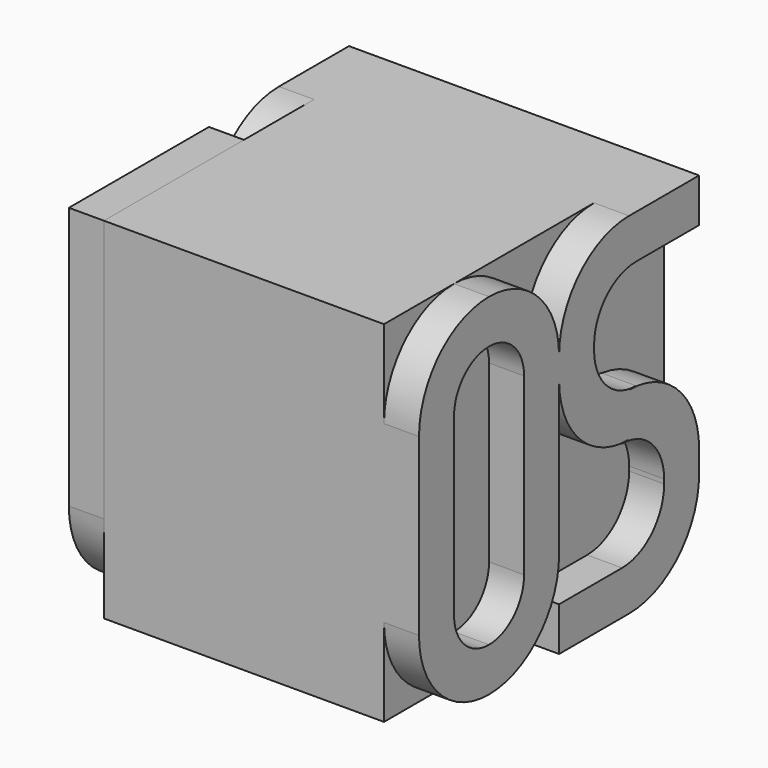
from build123d import *

# Parameters (mm, degrees)
F3_DEPTH = 2.54
F4_DEPTH = 2.54
F5_W     = 25.4
F5_H     = 25.4
F6_DEPTH = 20.32


with BuildPart() as f3:
    # F0 (on Right) → F3 (new body)
    with BuildSketch(Plane.YZ):
        with BuildLine():
            Line((0, 4.7625), (0, 6.35))
            ThreePointArc((0, 6.35), (-1.8598719395, 10.8401280605), (-6.35, 12.7))
            ThreePointArc((-6.35, 12.7), (-10.8401280605, 10.8401280605), (-12.7, 6.35))
            Line((-12.7, 6.35), (-12.7, -6.35))
            ThreePointArc((-12.7, -6.35), (-10.8401280605, -10.8401280605), (-6.35, -12.7))
            ThreePointArc((-6.35, -12.7), (-1.8598719395, -10.8401280605), (0, -6.35))
            Line((0, -6.35), (0, -3.81))
            Line((0, -3.81), (0, 4.7625))
        make_face()
        with BuildLine():
            ThreePointArc((-6.35, 9.525), (-4.1049359697, 8.5950640303), (-3.175, 6.35))
            Line((-3.175, 6.35), (-3.175, -6.35))
            ThreePointArc((-3.175, -6.35), (-4.1049359697, -8.5950640303), (-6.35, -9.525))
            ThreePointArc((-6.35, -9.525), (-8.5950640303, -8.5950640303), (-9.525, -6.35))
            Line((-9.525, -6.35), (-9.525, 6.35))
            ThreePointArc((-9.525, 6.35), (-8.5950640303, 8.5950640303), (-6.35, 9.525))
        make_face(mode=Mode.SUBTRACT)
        with BuildLine():
            Line((12.7, 12.7), (11.43, 12.7))
            Line((11.43, 12.7), (6.35, 12.7))
            ThreePointArc((6.35, 12.7), (1.8598719395, 10.8401280605), (0, 6.35))
            Line((0, 6.35), (0, 4.7625))
            ThreePointArc((0, 4.7625), (1.8598719395, 0.2723719395), (6.35, -1.5875))
            Line((6.35, -1.5875), (5.715, -1.5875))
            ThreePointArc((5.715, -1.5875), (8.4090768363, -2.7034231637), (9.525, -5.3975))
            Line((9.525, -5.3975), (9.525, -5.715))
            ThreePointArc((9.525, -5.715), (8.4090768363, -8.4090768363), (5.715, -9.525))
            Line((5.715, -9.525), (1.27, -9.525))
            Line((1.27, -9.525), (0, -9.525))
            Line((0, -9.525), (0, -12.7))
            Line((0, -12.7), (1.27, -12.7))
            Line((1.27, -12.7), (6.35, -12.7))
            ThreePointArc((6.35, -12.7), (10.8401280605, -10.8401280605), (12.7, -6.35))
            Line((12.7, -6.35), (12.7, -4.7625))
            ThreePointArc((12.7, -4.7625), (10.8401280605, -0.2723719395), (6.35, 1.5875))
            Line((6.35, 1.5875), (6.985, 1.5875))
            ThreePointArc((6.985, 1.5875), (4.2909231637, 2.7034231637), (3.175, 5.3975))
            Line((3.175, 5.3975), (3.175, 5.715))
            ThreePointArc((3.175, 5.715), (4.2909231637, 8.4090768363), (6.985, 9.525))
            Line((6.985, 9.525), (11.43, 9.525))
            Line((11.43, 9.525), (12.7, 9.525))
            Line((12.7, 9.525), (12.7, 12.7))
        make_face()
    extrude(amount=F3_DEPTH)



with BuildPart() as f4:
    # F2 (on offset) → F4 (new body)
    with BuildSketch(Plane.YZ.offset(-20.32)):
        with BuildLine():
            Line((12.7, -12.7), (12.7, 12.7))
            Line((12.7, 12.7), (6.35, 12.7))
            ThreePointArc((6.35, 12.7), (1.8598719395, 10.8401280605), (0, 6.35))
            ThreePointArc((0, 6.35), (1.8598719395, 1.8598719395), (6.35, 0))
            ThreePointArc((6.35, 0), (1.8598719395, -1.8598719395), (0, -6.35))
            ThreePointArc((0, -6.35), (1.8598719395, -10.8401280605), (6.35, -12.7))
            Line((6.35, -12.7), (12.7, -12.7))
        make_face()
        with BuildLine():
            Line((9.525, -2.54), (9.525, -9.525))
            Line((9.525, -9.525), (6.35, -9.525))
            ThreePointArc((6.35, -9.525), (4.1049359697, -8.5950640303), (3.175, -6.35))
            Line((3.175, -6.35), (3.175, -5.715))
            ThreePointArc((3.175, -5.715), (4.1049359697, -3.4699359697), (6.35, -2.54))
            Line((6.35, -2.54), (9.525, -2.54))
        make_face(mode=Mode.SUBTRACT)
        with BuildLine():
            Line((6.35, 9.525), (9.525, 9.525))
            Line((9.525, 9.525), (9.525, 2.54))
            Line((9.525, 2.54), (6.35, 2.54))
            ThreePointArc((6.35, 2.54), (4.1049359697, 3.4699359697), (3.175, 5.715))
            Line((3.175, 5.715), (3.175, 6.35))
            ThreePointArc((3.175, 6.35), (4.1049359697, 8.5950640303), (6.35, 9.525))
        make_face(mode=Mode.SUBTRACT)
    extrude(amount=-F4_DEPTH)


with BuildPart() as f4b:
    # F2 (on offset) → F4, piece 2 (new body)
    with BuildSketch(Plane.YZ.offset(-20.32)):
        with BuildLine():
            ThreePointArc((-6.35, -12.7), (-1.8598719395, -10.8401280605), (0, -6.35))
            Line((0, -6.35), (0, -5.7529052719))
            Line((0, -5.7529052719), (-3.175, -5.7529052719))
            Line((-3.175, -5.7529052719), (-3.175, -6.35))
            ThreePointArc((-3.175, -6.35), (-4.1049359697, -8.5950640303), (-6.35, -9.525))
            ThreePointArc((-6.35, -9.525), (-8.5950640303, -8.5950640303), (-9.525, -6.35))
            Line((-9.525, -6.35), (-9.525, 9.525))
            Line((-9.525, 9.525), (0, 9.525))
            Line((0, 9.525), (0, 12.7))
            Line((0, 12.7), (-12.7, 12.7))
            Line((-12.7, 12.7), (-12.7, -6.35))
            ThreePointArc((-12.7, -6.35), (-10.8401280605, -10.8401280605), (-6.35, -12.7))
        make_face()
    extrude(amount=-F4_DEPTH)


with BuildPart() as f3_1:
    add(f3.part)

    add(f4.part)  # F6 merges F4
    # F5 (on face) → F6 (join)
    with BuildSketch(Plane.YZ.offset(-20.32)):
        Rectangle(F5_W, F5_H)
    extrude(amount=F6_DEPTH)


solid = Compound([f4b.part, f3_1.part])
